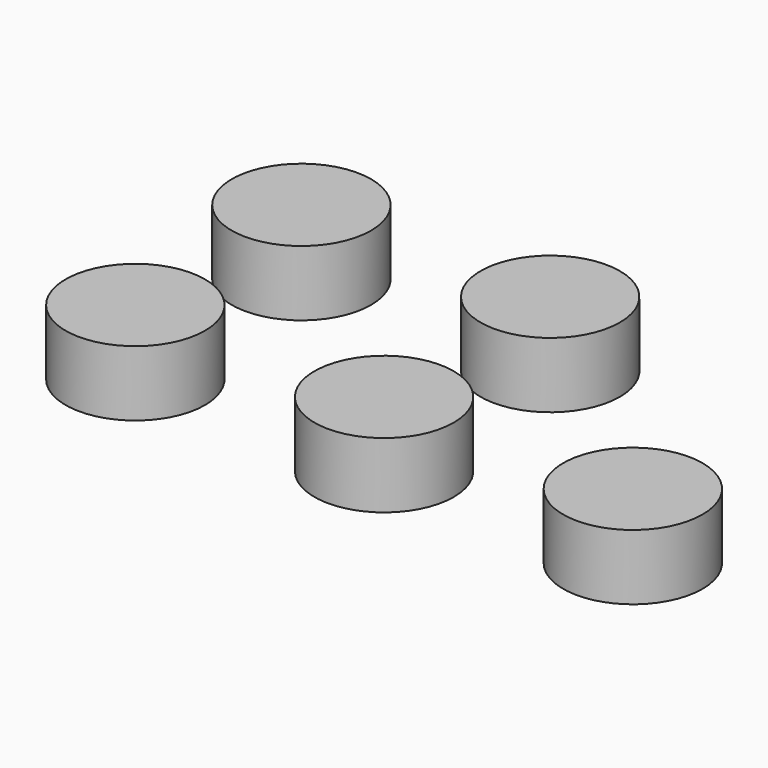
from build123d import *

# Parameters (mm, degrees)
F0_W       = 300
F0_H       = 160
F1_DEPTH   = 25
F2_W       = 300
F2_H       = 160
F2_R       = 26.6064560027
F1_FACE1_W = 300
F1_FACE1_H = 160
F3_DEPTH   = 25.001


with BuildPart() as f1:
    # F0 (on Top) → F1 (new body)
    with BuildSketch(Plane.XY):
        with Locations((3.7808977067, 9.5366072031)):
            Rectangle(F0_W, F0_H)
    extrude(amount=F1_DEPTH)

    # F2 (on face) + F1_face1 (on face) → F3 (cut, through all)
    with BuildSketch(Plane(origin=(0, 0, 0), x_dir=(1, 0, 0), z_dir=(0, 0, -1))):
        with Locations((3.7808977067, -9.5366072031)):
            Rectangle(F2_W, F2_H)
        with Locations((-97.7264517546, -50.4464879632)):
            Circle(F2_R, mode=Mode.SUBTRACT)
        with Locations((-2.7264517546, -50.4464879632)):
            Circle(F2_R, mode=Mode.SUBTRACT)
        with Locations((92.2735482454, -50.4464879632)):
            Circle(F2_R, mode=Mode.SUBTRACT)
        with Locations((-96, 31)):
            Circle(F2_R, mode=Mode.SUBTRACT)
        with Locations((-1, 31)):
            Circle(F2_R, mode=Mode.SUBTRACT)
        with Locations((94, 31)):
            Circle(F2_R, mode=Mode.SUBTRACT)
        with Locations((92.2735482454, -50.4464879632)):
            Circle(F2_R)
    with BuildSketch(Plane(origin=(3.7808977067, 9.5366072031, 25), x_dir=(1, 0, 0), z_dir=(0, 0, 1))):
        Rectangle(F1_FACE1_W, F1_FACE1_H)
    extrude(amount=-F3_DEPTH, dir=(0, 0, -1), mode=Mode.SUBTRACT)


solid = f1.part
